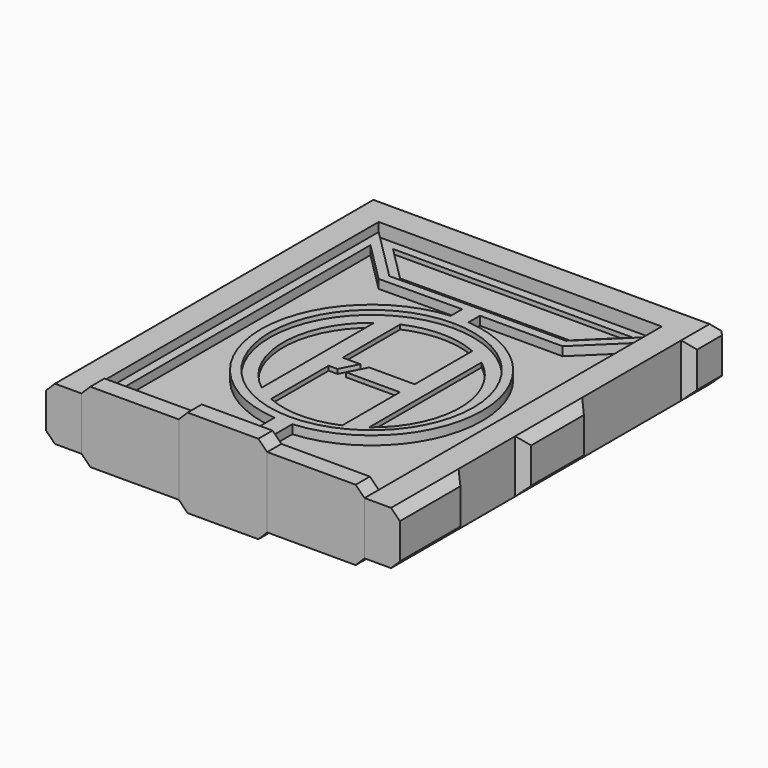
from build123d import *

# Parameters (mm, degrees)
F1_DEPTH       = 3
F2_DEPTH       = 4
F3_DEPTH       = 4
F4_DEPTH       = 5
F5_DEPTH       = 2
F6_DEPTH       = 1.5
F7_DEPTH       = 1.5
F8_DEPTH       = 1
F9_DEPTH       = 1
F10_DEPTH      = 1
F11_DEPTH      = 1
F12_DEPTH      = 1
F13_DEPTH      = 1
F14_SIZE       = 0.5
F15_SIZE       = 1
F16_DEPTH      = 1
F17_DEPTH      = 1.5
F17_DEPTH_BACK = 1
F18_DEPTH      = 1.5
F19_DEPTH      = 1.5
F19_DEPTH_BACK = 1


# Not quite as in the source:
# - ends of sketch curves that miss each other by under 0.0002 mm in the source are joined


with BuildPart() as f1:
    # F0 (on Top) → F1 (new body, symmetric)
    with BuildSketch(Plane.XY):
        Polygon((-15.9999780837, -19), (-16, 21), (16, 21), (15.9999777706, -19), (16, -21), (20, -21), (20, -12.4599365724), (19, -11.4606762967), (19, -3.4606762967), (20, -2.4606762967), (20, 4.9992602756), (19, 5.9992602756), (19, 19.9992586084), (20, 20.9992580527), (20, 25), (10.3202099967, 25), (9.3202099967, 24), (-9.4105946404, 24), (-10.4105946404, 25), (-20, 25), (-20, 20.9999978084), (-19, 19.9999983563), (-19, 6), (-20, 5), (-20, -2.4606762967), (-19, -3.4606762967), (-19, -11.4606762967), (-20, -12.1951649061), (-20, -21), (-16, -21), align=None)
    extrude(amount=F1_DEPTH, both=True)

    # F14
    f14_edges = [f1.edges().sort_by_distance(p)[0] for p in [
        (20, 25, 0),
        (-20, 25, 0),
    ]]
    chamfer(f14_edges, length=F14_SIZE)

    # F15 (call 1 of 24: OpenCascade refuses the feature's edges together)
    f15_edges = [f1.edges().sort_by_distance(p)[0] for p in [
        (20, 22.749629, 3),
    ]]
    chamfer(f15_edges, length=F15_SIZE)

    # F15#2 (call 2 of 24)
    f15_2_edges = [f1.edges().sort_by_distance(p)[0] for p in [
        (14.910105, 25, 3),
    ]]
    chamfer(f15_2_edges, length=F15_SIZE)

    # F15#3 (call 3 of 24)
    f15_3_edges = [f1.edges().sort_by_distance(p)[0] for p in [
        (20, 1.269292, 3),
    ]]
    chamfer(f15_3_edges, length=F15_SIZE)

    # F15#4 (call 4 of 24)
    f15_4_edges = [f1.edges().sort_by_distance(p)[0] for p in [
        (20, -16.729968, 3),
    ]]
    chamfer(f15_4_edges, length=F15_SIZE)

    # F15#5 (call 5 of 24)
    f15_5_edges = [f1.edges().sort_by_distance(p)[0] for p in [
        (-14.955297, 25, 3),
    ]]
    chamfer(f15_5_edges, length=F15_SIZE)

    # F15#6 (call 6 of 24)
    f15_6_edges = [f1.edges().sort_by_distance(p)[0] for p in [
        (-20, 22.749999, 3),
    ]]
    chamfer(f15_6_edges, length=F15_SIZE)

    # F15#7 (call 7 of 24)
    f15_7_edges = [f1.edges().sort_by_distance(p)[0] for p in [
        (-20, 1.269662, 3),
    ]]
    chamfer(f15_7_edges, length=F15_SIZE)

    # F15#8 (call 8 of 24)
    f15_8_edges = [f1.edges().sort_by_distance(p)[0] for p in [
        (-20, -16.597582, 3),
    ]]
    chamfer(f15_8_edges, length=F15_SIZE)

    # F15#9 (call 9 of 24)
    f15_9_edges = [f1.edges().sort_by_distance(p)[0] for p in [
        (20, -16.729968, -3),
    ]]
    chamfer(f15_9_edges, length=F15_SIZE)

    # F15#10 (call 10 of 24)
    f15_10_edges = [f1.edges().sort_by_distance(p)[0] for p in [
        (20, 1.269292, -3),
    ]]
    chamfer(f15_10_edges, length=F15_SIZE)

    # F15#11 (call 11 of 24)
    f15_11_edges = [f1.edges().sort_by_distance(p)[0] for p in [
        (20, 22.749629, -3),
    ]]
    chamfer(f15_11_edges, length=F15_SIZE)

    # F15#12 (call 12 of 24)
    f15_12_edges = [f1.edges().sort_by_distance(p)[0] for p in [
        (14.910105, 25, -3),
    ]]
    chamfer(f15_12_edges, length=F15_SIZE)

    # F15#13 (call 13 of 24)
    f15_13_edges = [f1.edges().sort_by_distance(p)[0] for p in [
        (-14.955297, 25, -3),
    ]]
    chamfer(f15_13_edges, length=F15_SIZE)

    # F15#14 (call 14 of 24)
    f15_14_edges = [f1.edges().sort_by_distance(p)[0] for p in [
        (-20, 22.749999, -3),
    ]]
    chamfer(f15_14_edges, length=F15_SIZE)

    # F15#15 (call 15 of 24)
    f15_15_edges = [f1.edges().sort_by_distance(p)[0] for p in [
        (-20, 1.269662, -3),
    ]]
    chamfer(f15_15_edges, length=F15_SIZE)

    # F15#16 (call 16 of 24)
    f15_16_edges = [f1.edges().sort_by_distance(p)[0] for p in [
        (-20, -16.597582, -3),
    ]]
    chamfer(f15_16_edges, length=F15_SIZE)


with BuildPart() as f2:
    # F0 (on Top) → F2 (new body, symmetric)
    with BuildSketch(Plane.XY):
        Polygon((-5, -19), (-15.9999780837, -19), (-16, -21), (-14, -21), (-5, -21), align=None)
    extrude(amount=F2_DEPTH, both=True)

    # F15#23 (call 23 of 24)
    f15_23_edges = [f2.edges().sort_by_distance(p)[0] for p in [
        (-15.999989, -20, 4),
    ]]
    chamfer(f15_23_edges, length=F15_SIZE)

    # F15#24 (call 24 of 24)
    f15_24_edges = [f2.edges().sort_by_distance(p)[0] for p in [
        (-15.999989, -20, -4),
    ]]
    chamfer(f15_24_edges, length=F15_SIZE)


with BuildPart() as f3:
    # F0 (on Top) → F3 (new body, symmetric)
    with BuildSketch(Plane.XY):
        Polygon((16, -21), (15.9999777706, -19), (5, -19), (5, -21), (14, -21), align=None)
    extrude(amount=F3_DEPTH, both=True)

    # F15#17 (call 17 of 24)
    f15_17_edges = [f3.edges().sort_by_distance(p)[0] for p in [
        (15.999989, -20, 4),
    ]]
    chamfer(f15_17_edges, length=F15_SIZE)

    # F15#18 (call 18 of 24)
    f15_18_edges = [f3.edges().sort_by_distance(p)[0] for p in [
        (15.999989, -20, -4),
    ]]
    chamfer(f15_18_edges, length=F15_SIZE)


with BuildPart() as f4:
    # F0 (on Top) → F4 (new body, symmetric)
    with BuildSketch(Plane.XY):
        Polygon((0, -19), (-5, -19), (-5, -21), (0, -21), (5, -21), (5, -19), align=None)
    extrude(amount=F4_DEPTH, both=True)

    # F15#19 (call 19 of 24)
    f15_19_edges = [f4.edges().sort_by_distance(p)[0] for p in [
        (5, -20, 5),
    ]]
    chamfer(f15_19_edges, length=F15_SIZE)

    # F15#20 (call 20 of 24)
    f15_20_edges = [f4.edges().sort_by_distance(p)[0] for p in [
        (-5, -20, 5),
    ]]
    chamfer(f15_20_edges, length=F15_SIZE)

    # F15#21 (call 21 of 24)
    f15_21_edges = [f4.edges().sort_by_distance(p)[0] for p in [
        (5, -20, -5),
    ]]
    chamfer(f15_21_edges, length=F15_SIZE)

    # F15#22 (call 22 of 24)
    f15_22_edges = [f4.edges().sort_by_distance(p)[0] for p in [
        (-5, -20, -5),
    ]]
    chamfer(f15_22_edges, length=F15_SIZE)


with BuildPart() as f5:
    # F0 (on Top) → F5 (new body, symmetric)
    with BuildSketch(Plane.XY):
        with BuildLine():
            Line((15.9999777706, -19), (16, 21))
            Line((16, 21), (9.9143997954, 15.0870461175))
            Line((9.9143997954, 15.0870461175), (-0.0184291639, 15.0870461175))
            Line((-0.0184291639, 15.0870461175), (-0.0184291639, 11.4999860088))
            ThreePointArc((-0.0184291639, 11.4999860088), (11.4999970838, 0.0092145849), (0, -11.5000007755))
            Line((0, -11.5000007755), (0, -19))
            Line((0, -19), (5, -19))
            Line((5, -19), (15.9999777706, -19))
        make_face()
        with BuildLine():
            Line((1, -18), (1, -12.4599365724))
            ThreePointArc((1, -12.4599365724), (12.4999973577, 0.0092436648), (0.9815708361, 12.4614019308))
            Line((0.9815708361, 12.4614019308), (0.9815708361, 14.0870461175))
            Line((0.9815708361, 14.0870461175), (10.3202099967, 14.0870461175))
            Line((10.3202099967, 14.0870461175), (14.9999986852, 18.6340708586))
            Line((14.9999986852, 18.6340708586), (14.9999783263, -18))
            Line((14.9999783263, -18), (1, -18))
        make_face(mode=Mode.SUBTRACT)
        with BuildLine():
            Line((-9.9999997795, 14.9999997795), (-16, 21))
            Line((-16, 21), (-15.9999780837, -19))
            Line((-15.9999780837, -19), (-5, -19))
            Line((-5, -19), (0, -19))
            Line((0, -19), (0, -11.5000007755))
            ThreePointArc((0, -11.5000007755), (-11.5092068117, -0.0092223522), (-0.0184291639, 11.4999852338))
            Line((-0.0184291639, 11.4999852338), (-0.0184291639, 15.0870461175))
            Line((-0.0184291639, 15.0870461175), (-9.9999997795, 14.9999997795))
        make_face()
        with BuildLine():
            ThreePointArc((-1.0184291639, 12.4591816806), (-12.5092070852, -0.0092519812), (-1, -12.4606762967))
            Line((-1, -12.4606762967), (-1, -18))
            Line((-1, -18), (-14.9999786316, -18))
            Line((-14.9999786316, -18), (-14.9999986772, 18.5857851149))
            Line((-14.9999986772, 18.5857851149), (-10.4105946404, 13.996381078))
            Line((-10.4105946404, 13.996381078), (-1.0184291639, 14.0782873873))
            Line((-1.0184291639, 14.0782873873), (-1.0184291639, 12.4591816806))
        make_face(mode=Mode.SUBTRACT)
    extrude(amount=F5_DEPTH, both=True)

    # F0 (on Top) → F7 (join, symmetric)
    with BuildSketch(Plane.XY):
        with BuildLine():
            ThreePointArc((0, -11.5000007755), (11.4999970838, 0.0092145849), (-0.0184291639, 11.4999860088))
            ThreePointArc((-0.0184291639, 11.4999860088), (-11.5092068117, -0.0092223522), (0, -11.5000007755))
        make_face()
        with BuildLine():
            Line((-6.0710678119, 7.9462025914), (-6.0710678119, 1))
            Line((-6.0710678119, 1), (-6.0710678119, -7.9462025914))
            ThreePointArc((-6.0710678119, -7.9462025914), (-10, 0), (-6.0710678119, 7.9462025914))
        make_face(mode=Mode.SUBTRACT)
        with BuildLine():
            Line((-2.0802817172, 0.9999922298), (-4.0710678119, 0.9999922298))
            Line((-4.0710678119, 0.9999922298), (-4.0710678119, 9.1338057167))
            ThreePointArc((-4.0710678119, 9.1338057167), (0, 10), (4.0710678119, 9.1338057167))
            Line((4.0710678119, 9.1338057167), (4.0710678119, 0.9999922298))
            Line((4.0710678119, 0.9999922298), (1.9906647528, 0.9999922298))
            Line((1.9906647528, 0.9999922298), (2.9906647528, -0.9994532542))
            Line((2.9906647528, -0.9994532542), (3.9906647528, -0.9994532542))
            Line((3.9906647528, -0.9994532542), (3.9906647528, -9.1332590577))
            ThreePointArc((3.9906647528, -9.1332590577), (-0.0481391757, -9.9706543084), (-4.0802817172, -9.1017501114))
            Line((-4.0802817172, -9.1017501114), (-4.0802817172, -0.9682968661))
            Line((-4.0802817172, -0.9682968661), (-3.0803120527, -0.9760859632))
            Line((-3.0803120527, -0.9760859632), (-2.0802817172, 0.9999922298))
        make_face(mode=Mode.SUBTRACT)
        with BuildLine():
            Line((6.0710678119, -7.9462025914), (6.0710678119, 1))
            Line((6.0710678119, 1), (6.0710678119, 7.9462025914))
            ThreePointArc((6.0710678119, 7.9462025914), (10, 0), (6.0710678119, -7.9462025914))
        make_face(mode=Mode.SUBTRACT)
    extrude(amount=F7_DEPTH, both=True)

    # F0 (on Top) → F9 (join, symmetric)
    with BuildSketch(Plane.XY):
        with BuildLine():
            Line((-1, -18), (-1, -12.4606762967))
            ThreePointArc((-1, -12.4606762967), (-12.5092070852, -0.0092519812), (-1.0184291639, 12.4591816806))
            Line((-1.0184291639, 12.4591816806), (-1.0184291639, 14.0782873873))
            Line((-1.0184291639, 14.0782873873), (-10.4105946404, 13.996381078))
            Line((-10.4105946404, 13.996381078), (-14.9999986772, 18.5857851149))
            Line((-14.9999986772, 18.5857851149), (-14.9999786316, -18))
            Line((-14.9999786316, -18), (-1, -18))
        make_face()
    extrude(amount=F9_DEPTH, both=True)

    # F0 (on Top) → F10 (join, symmetric)
    with BuildSketch(Plane.XY):
        with BuildLine():
            ThreePointArc((0.9815708361, 12.4614019308), (12.4999973577, 0.0092436648), (1, -12.4599365724))
            Line((1, -12.4599365724), (1, -18))
            Line((1, -18), (14.9999783263, -18))
            Line((14.9999783263, -18), (14.9999986852, 18.6340708586))
            Line((14.9999986852, 18.6340708586), (10.3202099967, 14.0870461175))
            Line((10.3202099967, 14.0870461175), (0.9815708361, 14.0870461175))
            Line((0.9815708361, 14.0870461175), (0.9815708361, 12.4614019308))
        make_face()
    extrude(amount=F10_DEPTH, both=True)

    # F0 (on Top) → F11 (join, symmetric)
    with BuildSketch(Plane.XY):
        with BuildLine():
            Line((-6.0710678119, -7.9462025914), (-6.0710678119, 1))
            Line((-6.0710678119, 1), (-6.0710678119, 7.9462025914))
            ThreePointArc((-6.0710678119, 7.9462025914), (-10, 0), (-6.0710678119, -7.9462025914))
        make_face()
    extrude(amount=F11_DEPTH, both=True)

    # F0 (on Top) → F12 (join, symmetric)
    with BuildSketch(Plane.XY):
        with BuildLine():
            Line((-4.0710678119, 9.1338057167), (-4.0710678119, 0.9999922298))
            Line((-4.0710678119, 0.9999922298), (-2.0802817172, 0.9999922298))
            Line((-2.0802817172, 0.9999922298), (-1.0802817172, 0.9999922298))
            Line((-1.0802817172, 0.9999922298), (-0.0092139053, 0.9999922298))
            Line((-0.0092139053, 0.9999922298), (0.9906647528, 0.9999922298))
            Line((0.9906647528, 0.9999922298), (1.9906647528, 0.9999922298))
            Line((1.9906647528, 0.9999922298), (4.0710678119, 0.9999922298))
            Line((4.0710678119, 0.9999922298), (4.0710678119, 9.1338057167))
            ThreePointArc((4.0710678119, 9.1338057167), (0, 10), (-4.0710678119, 9.1338057167))
        make_face()
    extrude(amount=F12_DEPTH, both=True)

    # F0 (on Top) → F13 (join, symmetric)
    with BuildSketch(Plane.XY):
        with BuildLine():
            Line((6.0710678119, 7.9462025914), (6.0710678119, 1))
            Line((6.0710678119, 1), (6.0710678119, -7.9462025914))
            ThreePointArc((6.0710678119, -7.9462025914), (10, 0), (6.0710678119, 7.9462025914))
        make_face()
    extrude(amount=F13_DEPTH, both=True)

    # F0 (on Top) → F16 (join, symmetric)
    with BuildSketch(Plane.XY):
        with BuildLine():
            Line((-2.0803423881, -0.9838750602), (-3.0803120527, -0.9760859632))
            Line((-3.0803120527, -0.9760859632), (-4.0802817172, -0.9682968661))
            Line((-4.0802817172, -0.9682968661), (-4.0802817172, -9.1017501114))
            ThreePointArc((-4.0802817172, -9.1017501114), (-0.0481391757, -9.9706543084), (3.9906647528, -9.1332590577))
            Line((3.9906647528, -9.1332590577), (3.9906647528, -0.9994532542))
            Line((3.9906647528, -0.9994532542), (2.9906647528, -0.9994532542))
            Line((2.9906647528, -0.9994532542), (1.9906647528, -0.9994532542))
            Line((1.9906647528, -0.9994532542), (0.9906647528, -0.9994532542))
            Line((0.9906647528, -0.9994532542), (-0.0804030591, -0.9994532542))
            Line((-0.0804030591, -0.9994532542), (-2.0803423881, -0.9838750602))
        make_face()
    extrude(amount=F16_DEPTH, both=True)

    # F0 (on Top) → F17 (join, two sides)
    with BuildSketch(Plane.XY) as f17_sk:
        Polygon((-1.0802817172, 0.9999922298), (-2.0802817172, 0.9999922298), (-3.0803120527, -0.9760859632), (-2.0803423881, -0.9838750602), align=None)
    extrude(amount=-F17_DEPTH)
    extrude(f17_sk.sketch, amount=F17_DEPTH_BACK)

    # F0 (on Top) → F18 (join, symmetric)
    with BuildSketch(Plane.XY):
        Polygon((-0.0092139053, 0.9999922298), (-1.0802817172, 0.9999922298), (-2.0803423881, -0.9838750602), (-0.0804030591, -0.9994532542), (0.9906647528, -0.9994532542), (1.9906647528, -0.9994532542), (0.9906647528, 0.9999922298), align=None)
    extrude(amount=F18_DEPTH, both=True)

    # F0 (on Top) → F19 (join, two sides)
    with BuildSketch(Plane.XY) as f19_sk:
        Polygon((2.9906647528, -0.9994532542), (1.9906647528, 0.9999922298), (0.9906647528, 0.9999922298), (1.9906647528, -0.9994532542), align=None)
    extrude(amount=F19_DEPTH)
    extrude(f19_sk.sketch, amount=-F19_DEPTH_BACK)


with BuildPart() as f6:
    # F0 (on Top) → F6 (new body, symmetric)
    with BuildSketch(Plane.XY):
        Polygon((16, 21), (-16, 21), (-9.9999997795, 14.9999997795), (-0.0184291639, 15.0870461175), (9.9143997954, 15.0870461175), align=None)
        Polygon((-9.5857864376, 16), (-13.5857864376, 20), (13.5357938344, 20), (9.5146165577, 16.0929020982), align=None, mode=Mode.SUBTRACT)
    extrude(amount=F6_DEPTH, both=True)

    # F0 (on Top) → F8 (join, symmetric)
    with BuildSketch(Plane.XY):
        Polygon((13.5357938344, 20), (-13.5857864376, 20), (-9.5857864376, 16), (9.5146165577, 16.0929020982), align=None)
    extrude(amount=F8_DEPTH, both=True)


solid = Compound([f1.part, f2.part, f3.part, f4.part, f5.part, f6.part])
